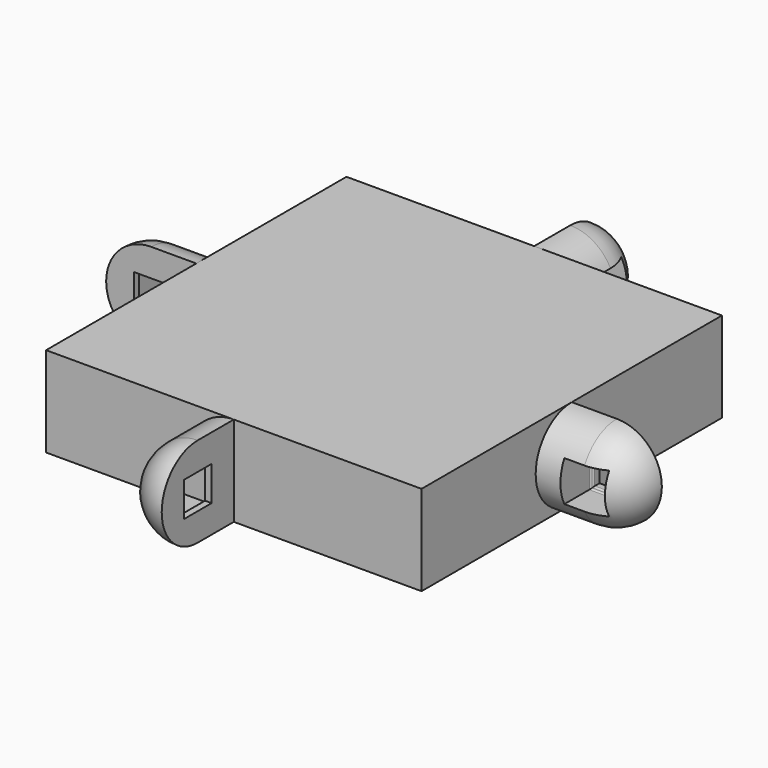
from build123d import *

# Parameters (mm, degrees)
F0_W      = 50
F0_H      = 50
F1_DEPTH  = 12
F3_DEPTH  = 12
F5_W      = 7.196964696
F5_H      = 12
F6_DEPTH  = 25
F7_W      = 5.4
F7_H      = 5.4
F8_DEPTH  = 25
F9_W      = 5.4
F9_H      = 5.4
F9_W_2    = 4.6
F9_H_2    = 4.6
F10_DEPTH = 1
F11_R     = 0.19999
F13_W     = 25
F13_H     = 12
F14_DEPTH = 50
F15_W     = 25
F15_H     = 12
F16_DEPTH = 25
F17_COUNT = 4


# Not quite as in the source:
# - a fillet or chamfer that OpenCascade refuses, or shapes differently, is made with other operations: its cross-section is extruded or revolved along the edge and cut away or added
# - a fillet or chamfer is up to 0.001 mm smaller than in the source, because OpenCascade refuses the exact size


with BuildPart() as f1:
    # F0 (on Top) → F1 (new body)
    with BuildSketch(Plane.XY):
        Rectangle(F0_W, F0_H)
    extrude(amount=F1_DEPTH)

    # F2 (on face) → F3 (join)
    with BuildSketch(Plane(origin=(-25, 0, 0), x_dir=(0, -1, 0), z_dir=(-1, 0, 0))):
        with BuildLine():
            ThreePointArc((0, 0), (4.2426406871, 1.7573593129), (6, 6))
            ThreePointArc((6, 6), (4.2426406871, 10.2426406871), (0, 12))
            ThreePointArc((0, 12), (-6, 6), (0, 0))
        make_face()
    extrude(amount=F3_DEPTH)

    # F4: fillet of radius 6 on 1 edges, made by hand

    # F4_s1 → F4_t2 (revolve, cut)
    with BuildSketch(Plane.XZ):
        with BuildLine():
            ThreePointArc((-31, 12), (-35.2426406871, 10.2426406871), (-37, 6))
            Line((-37, 6), (-37.12, 6))
            Line((-37.12, 6), (-37.12, 12.12))
            Line((-37.12, 12.12), (-31, 12.12))
            Line((-31, 12.12), (-31, 12))
        make_face()
    revolve(axis=Axis((-37, 0, 6), (1, 0, 0)), mode=Mode.SUBTRACT)

    # F5 (on face) → F6 (cut)
    with BuildSketch(Plane(origin=(-25, 0, 0), x_dir=(0, -1, 0), z_dir=(-1, 0, 0))):
        with Locations((3.598482348, 6)):
            Rectangle(F5_W, F5_H)
    extrude(amount=F6_DEPTH, mode=Mode.SUBTRACT)

    # F7 (on face) → F8 (cut)
    with BuildSketch(Plane.XZ):
        with Locations((-31, 6)):
            Rectangle(F7_W, F7_H)
    extrude(amount=-F8_DEPTH, mode=Mode.SUBTRACT)

    # F9 (on face) → F10 (join)
    with BuildSketch(Plane.XZ):
        with Locations((-31, 6)):
            Rectangle(F9_W, F9_H)
        with Locations((-31, 6)):
            Rectangle(F9_W_2, F9_H_2, mode=Mode.SUBTRACT)
    extrude(amount=-F10_DEPTH)

    # F11 (radius 0.2 in the source; OpenCascade refuses exactly that, so slightly less here)
    f11_edges = [f1.edges().sort_by_distance(p)[0] for p in [
        (-28.7, 1, 6),
        (-28.3, 1, 6),
        (-31, 1, 8.7),
        (-31, 1, 8.3),
        (-33.7, 1, 6),
        (-33.3, 1, 6),
        (-31, 1, 3.3),
        (-31, 1, 3.7),
    ]]
    fillet(f11_edges, radius=F11_R)

    # F13 (on face) → F14 (cut)
    with BuildSketch(Plane(origin=(-25, 0, 0), x_dir=(0, -1, 0), z_dir=(-1, 0, 0))):
        with Locations((12.5, 6)):
            Rectangle(F13_W, F13_H)
    extrude(amount=-F14_DEPTH, mode=Mode.SUBTRACT)

    # F15 (on face) → F16 (cut)
    with BuildSketch(Plane(origin=(0, 25, 0), x_dir=(-1, 0, 0), z_dir=(0, 1, 0))):
        with Locations((-12.5, 6)):
            Rectangle(F15_W, F15_H)
    extrude(amount=-F16_DEPTH, mode=Mode.SUBTRACT)

    # F17: F1 ×4 about axis
    f17_axis = Axis((0, 0, 13.6458836496), (0, 0, 1))


with BuildPart() as f1_1:
    add(f1.part)
    for i in range(1, F17_COUNT):
        add(f1.part.rotate(f17_axis, i * 360 / F17_COUNT))


solid = f1_1.part
